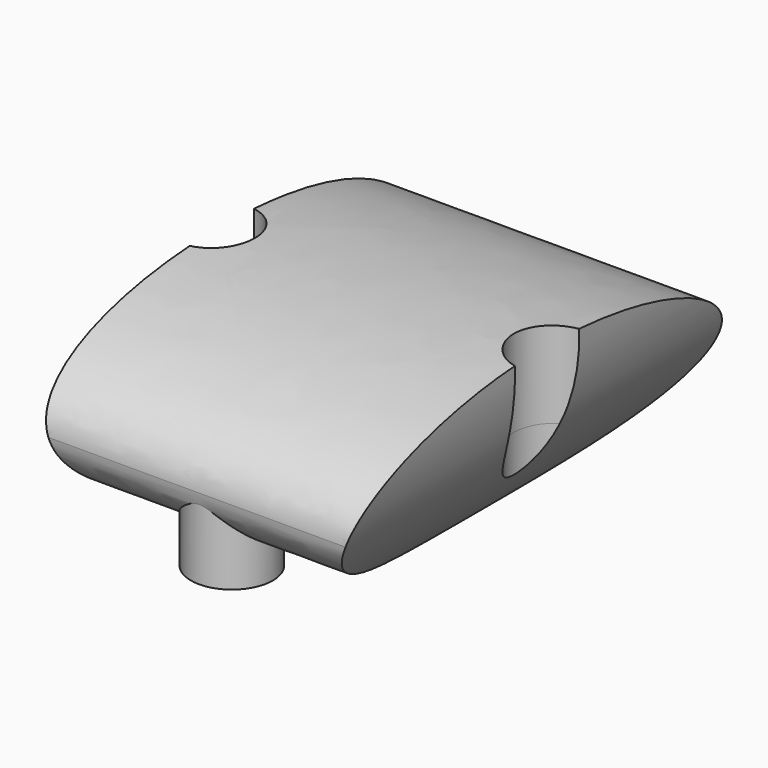
from build123d import *

# Parameters (mm, degrees)
F1_DEPTH      = 343
F3_START      = -239.0181699509
F3_DEPTH      = 477.7438594859
F6_R          = 60
F6_R_2        = 12.5
F7_DEPTH      = 120
F8_R          = 60
F9_DEPTH      = 127.5010001
F9_DEPTH_BACK = 127.5010001152


# Not quite as in the source:
# - a feature of the source that left no trace in its solid (it failed there, or was rolled back) is left out


with BuildPart() as f1:
    # F0 (on Front) → F1 (new body, symmetric)
    with BuildSketch(Plane.XZ):
        with BuildLine():
            Line((-127.808437634, -127.5), (127.808437634, -127.5))
            ThreePointArc((127.808437634, -127.5), (212.1294622405, -12.5777057431), (238.5, 127.5))
            Line((238.5, 127.5), (-238.5, 127.5))
            ThreePointArc((-238.5, 127.5), (-213.5093149969, -13.1766785173), (-127.808437634, -127.5))
        make_face()
    extrude(amount=F1_DEPTH, both=True)

    # F2 (on Right) → F3 (intersect)
    with BuildSketch(Plane.YZ.offset(F3_START)):
        with BuildLine():
            add(Edge.make_bspline(
                [(343, 0), (343, 220.836477965), (-171.5, 110.4182389825), (-686, 0), (-171.5, -110.4182389825), (343, -220.836477965), (343, 0)],
                knots=[0, 0, 0, 2.0943951024, 2.0943951024, 4.1887902048, 4.1887902048, 6.2831853072, 6.2831853072, 6.2831853072], degree=2, weights=[1, 0.5, 1, 0.5, 1, 0.5, 1]))
        make_face()
    extrude(amount=F3_DEPTH, mode=Mode.INTERSECT)

    # F5: F1 across face


with BuildPart() as f1_1:
    add(f1.part)
    add(f1.part.mirror(Plane.XZ))

    # F6 (on Top) → F7 (join)
    with BuildSketch(Plane.XY):
        with Locations((0, -280)):
            Circle(F6_R)
        with Locations((0, -280)):
            Circle(F6_R_2, mode=Mode.SUBTRACT)
    extrude(amount=-F7_DEPTH)

    # F8 (on Top) → F9 (cut, two sides)
    with BuildSketch(Plane.XY) as f9_sk:
        with Locations((-250, 0)):
            Circle(F8_R)
        with Locations((250, 0)):
            Circle(F8_R)
    extrude(amount=F9_DEPTH, mode=Mode.SUBTRACT)
    extrude(f9_sk.sketch, amount=-F9_DEPTH_BACK, mode=Mode.SUBTRACT)


solid = f1_1.part
